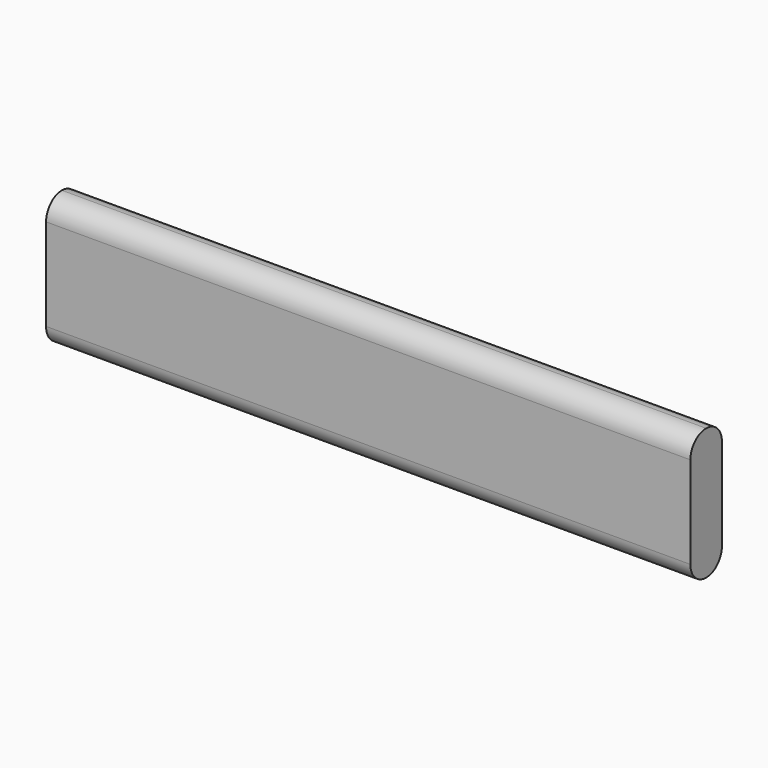
from build123d import *

# Parameters (mm, degrees)
F0_W     = 311.15
F0_H     = 63.5
F1_DEPTH = 19.05
F2_R     = 9.52499


# Not quite as in the source:
# - a fillet or chamfer is up to 0.001 mm smaller than in the source, because OpenCascade refuses the exact size


with BuildPart() as f1:
    # F0 (on Front) → F1 (new body)
    with BuildSketch(Plane.XZ):
        with Locations((155.575, 31.75)):
            Rectangle(F0_W, F0_H)
    extrude(amount=F1_DEPTH)

    # F2 (radius 9.525 in the source; OpenCascade refuses exactly that, so slightly less here)
    f2_edges = [f1.edges().sort_by_distance(p)[0] for p in [
        (155.575, -19.05, 63.5),
        (155.575, 0, 63.5),
        (155.575, -19.05, 0),
        (155.575, 0, 0),
    ]]
    fillet(f2_edges, radius=F2_R)


solid = f1.part
